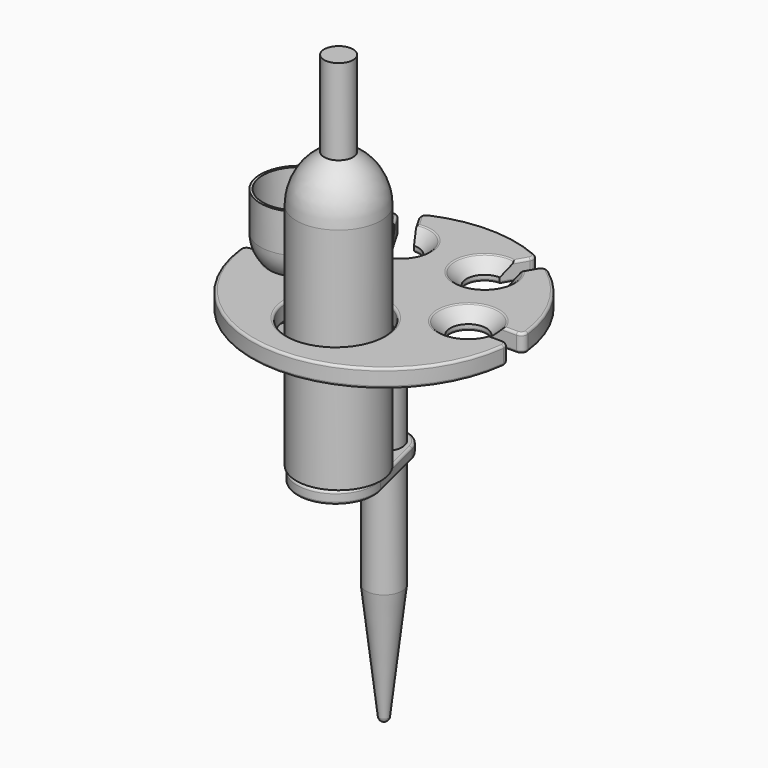
from build123d import *

# Parameters (mm, degrees)
F0_R            = 110
F0_R_2          = 40
F1_DEPTH        = 15
F3_DEPTH        = 15.001
F3_COPIES_COUNT = 4
F3_COPIES_ANGLE = 180
F5_SIZE         = 10
F6_R            = 5
F7_R            = 2
F11_R           = 15
F12_DEPTH       = 10
F13_R           = 2
F18_SIZE2       = 3
F18_SIZE        = 26


# Not quite as in the source:
# - a pattern or mirror of a feature is missing from the dataset's text; its kind, count and spacing are read off the source's solid


with BuildPart() as f1:
    # F0 (on Top) → F1 (new body)
    with BuildSketch(Plane.XY):
        Circle(F0_R)
        with Locations((0, -50)):
            Circle(F0_R_2, mode=Mode.SUBTRACT)
    extrude(amount=F1_DEPTH)

    # F2 (on Top) → F3 (cut, through all)
    with BuildSketch(Plane.XY):
        with BuildLine():
            Line((-128.2664991614, -7), (-83.2664991614, -7))
            ThreePointArc((-83.2664991614, -7), (-55, 0), (-83.2664991614, 7))
            Line((-83.2664991614, 7), (-128.2664991614, 7))
            Line((-128.2664991614, 7), (-128.2664991614, -7))
        make_face()
    f3 = extrude(amount=F3_DEPTH, mode=Mode.SUBTRACT)

    # F3_copies: F3 ×4 about axis
    f3_copies_axis = Axis((0, 0, 0), (0, 0, -1))
    for i in range(1, F3_COPIES_COUNT):
        add(f3.rotate(f3_copies_axis, i * F3_COPIES_ANGLE / (F3_COPIES_COUNT - 1)), mode=Mode.SUBTRACT)

    # F5
    f5_edges = [f1.edges().sort_by_distance(p)[0] for p in [
        (-55, 0, 15),
        (-27.5, 47.631397, 15),
        (27.5, 47.631397, 15),
        (55, 0, 15),
    ]]
    chamfer(f5_edges, length=F5_SIZE)

    # F6
    f6_edges = [f1.edges().sort_by_distance(p)[0] for p in [
        (-109.777047, 7, 7.5),
        (-109.777047, -7, 7.5),
        (109.777047, -7, 7.5),
        (-60.950701, 91.569711, 7.5),
        (-48.826346, 98.569711, 7.5),
        (48.826346, 98.569711, 7.5),
        (109.777047, 7, 7.5),
        (60.950701, 91.569711, 7.5),
    ]]
    fillet(f6_edges, radius=F6_R)

    # F7
    f7_edges = [f1.edges().sort_by_distance(p)[0] for p in [
        (-99.156016, 7, 15),
        (-108.044132, 8.672624, 15),
        (-45, 0, 15),
        (-95.262794, 55, 15),
        (-99.156016, -7, 15),
        (-61.532779, 89.232651, 15),
        (-108.044132, -8.672624, 15),
        (-55.640186, 82.371629, 15),
        (0, -110, 15),
        (-22.5, 38.971143, 15),
        (108.044132, -8.672624, 15),
        (-43.51583, 89.371629, 15),
        (99.156016, -7, 15),
        (-46.511353, 97.905275, 15),
        (45, 0, 15),
        (0, 110, 15),
        (99.156016, 7, 15),
        (46.511353, 97.905275, 15),
        (108.044132, 8.672624, 15),
        (43.51583, 89.371629, 15),
        (95.262794, 55, 15),
        (22.5, 38.971143, 15),
        (61.532779, 89.232651, 15),
        (55.640186, 82.371629, 15),
        (-40, -50, 15),
        (-93.789266, -7, 0),
        (-108.044132, -8.672624, 0),
        (-55, 0, 0),
        (0, -110, 0),
        (-93.789266, 7, 0),
        (108.044132, -8.672624, 0),
        (-108.044132, 8.672624, 0),
        (93.789266, -7, 0),
        (-95.262794, 55, 0),
        (55, 0, 0),
        (-61.532779, 89.232651, 0),
        (93.789266, 7, 0),
        (-52.956811, 77.723887, 0),
        (108.044132, 8.672624, 0),
        (-27.5, 47.631397, 0),
        (95.262794, 55, 0),
        (-40.832455, 84.723887, 0),
        (61.532779, 89.232651, 0),
        (-46.511353, 97.905275, 0),
        (52.956811, 77.723887, 0),
        (0, 110, 0),
        (27.5, 47.631397, 0),
        (46.511353, 97.905275, 0),
        (40.832455, 84.723887, 0),
        (-40, -50, 0),
    ]]
    fillet(f7_edges, radius=F7_R)

    # F8 (on Front) → F9 (revolve)
    with BuildSketch(Plane.XZ):
        with BuildLine():
            Line((0, -300), (0, 0))
            Line((0, 0), (-15, 0))
            Line((-15, 0), (-15, -200))
            Line((-15, -200), (-3.9741189123, -296.4542894134))
            ThreePointArc((-3.9741189123, -296.4542894134), (-2.6629722442, -298.9847242464), (0, -300))
        make_face()
    revolve(axis=Axis((0, 0, -150), (0, 0, -1)))

    # F11 (on offset) → F12 (join)
    with BuildSketch(Plane(origin=(0, 0, -95), x_dir=(1, 0, 0), z_dir=(0, 0, -1))):
        with BuildLine():
            Line((-31.0647324147, 42.32), (-19.4154577592, -4.8))
            ThreePointArc((-19.4154577592, -4.8), (0, -20), (19.4154577592, -4.8))
            Line((19.4154577592, -4.8), (31.0647324147, 42.32))
            ThreePointArc((31.0647324147, 42.32), (0, 82), (-31.0647324147, 42.32))
        make_face()
        Circle(F11_R, mode=Mode.SUBTRACT)
    extrude(amount=F12_DEPTH)

    # F13
    f13_edges = [f1.edges().sort_by_distance(p)[0] for p in [
        (0, -82, -95),
        (0, -82, -105),
        (25.240095, -18.76, -95),
        (-25.240095, -18.76, -95),
        (0, 20, -95),
        (0, 20, -105),
        (25.240095, -18.76, -105),
        (-25.240095, -18.76, -105),
    ]]
    fillet(f13_edges, radius=F13_R)


with BuildPart() as f15:
    # F14 (on Right) → F15 (revolve)
    with BuildSketch(Plane.YZ):
        with BuildLine():
            Line((-47, -94), (-12, -94))
            Line((-12, -94), (-12, 96))
            ThreePointArc((-12, 96), (-18.1782586535, 118.6384628453), (-35, 135))
            Line((-35, 135), (-35, 206))
            Line((-35, 206), (-47, 206))
            Line((-47, 206), (-47, -94))
        make_face()
    revolve(axis=Axis((0, -47, 56), (0, 0, -1)))


with BuildPart() as f17:
    # F16 (on Front) → F17 (revolve)
    with BuildSketch(Plane.XZ):
        with BuildLine():
            Line((-70, 8.0979797464), (-70, -48.9020202536))
            Line((-70, -48.9020202536), (-37.5, -48.9020202536))
            Line((-37.5, -48.9020202536), (-37.5, -44.9020202536))
            Line((-37.5, -44.9020202536), (-65.5, -44.9020202536))
            Line((-65.5, -44.9020202536), (-65.5, 6.0979797464))
            ThreePointArc((-65.5, 6.0979797464), (-45.7010101268, 14.2989898732), (-37.5, 34.0979797464))
            Line((-37.5, 34.0979797464), (-37.5, 66.0979797464))
            Line((-37.5, 66.0979797464), (-39.5, 66.0979797464))
            Line((-39.5, 66.0979797464), (-39.5, 34.0979797464))
            ThreePointArc((-39.5, 34.0979797464), (-47.1152236891, 15.7132034356), (-65.5, 8.0979797464))
            Line((-65.5, 8.0979797464), (-70, 8.0979797464))
        make_face()
    revolve(axis=Axis((-70, 0, -20.4020202536), (0, 0, -1)))

    # F18
    f18_edges = [f17.edges().sort_by_distance(p)[0] for p in [
        (-102.5, 0, -44.90202),
    ]]
    f18_side = f17.faces().sort_by_distance((-101.580761, 0, -44.90202))[0]
    chamfer(f18_edges, length=F18_SIZE, length2=F18_SIZE2, reference=f18_side)


solid = Compound([f1.part, f15.part, f17.part])
